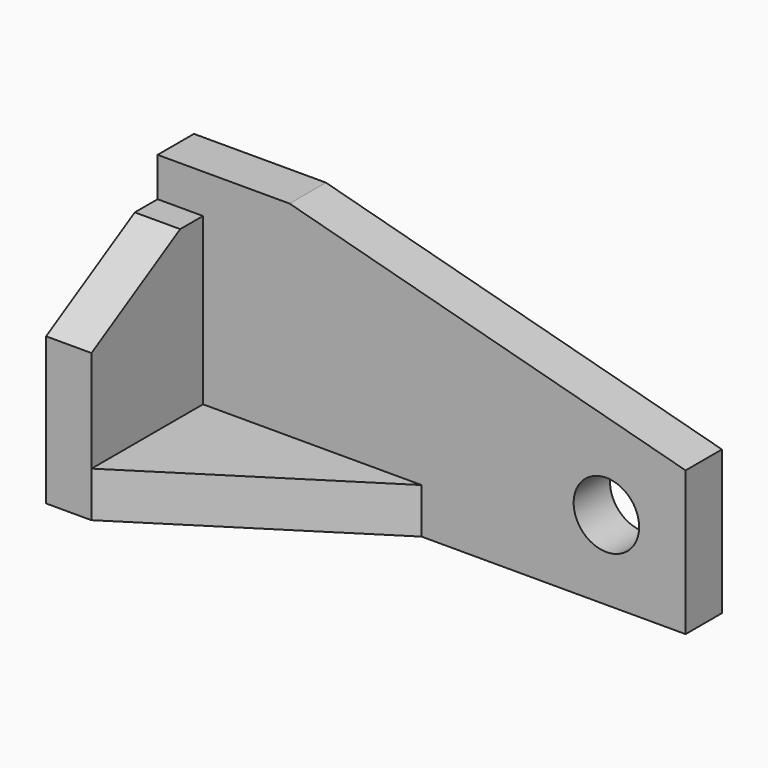
from build123d import *

# Parameters (mm, degrees)
F0_W     = 10.922
F0_H     = 28.702
F0_W_2   = 52.578
F0_H_2   = 10.922
F0_R     = 7.874
F1_DEPTH = 10.922
F2_DEPTH = 44.45
F3_SIZE2 = 52.628408
F3_SIZE  = 33.52799
F4_SIZE2 = 15.3979316793
F4_SIZE  = 26.67


# Not quite as in the source:
# - a fillet or chamfer is up to 0.001 mm smaller than in the source, because OpenCascade refuses the exact size


with BuildPart() as f1:
    # F0 (on Front) → F1 (new body)
    with BuildSketch(Plane.XZ):
        with Locations((-40.1902680954, 6.35)):
            Rectangle(F0_W, F0_H)
        with Locations((-8.4402680954, -24.638)):
            Rectangle(F0_W_2, F0_H_2)
        Polygon((-13.9012680954, 30.099), (-45.6512680954, 30.099), (-45.6512680954, 20.701), (-34.7292680954, 20.701), (-34.7292680954, -8.001), (-34.7292680954, -19.177), (17.8487319046, -19.177), (17.8487319046, -30.099), (81.3487319046, -30.099), (81.3487319046, 4.5768394209), align=None)
        with Locations((62.2987319046, -11.049)):
            Circle(F0_R, mode=Mode.SUBTRACT)
        Polygon((-34.7292680954, -8.001), (-45.6512680954, -8.001), (-45.6512680954, -30.099), (-34.7292680954, -30.099), (-34.7292680954, -19.177), align=None)
    extrude(amount=F1_DEPTH)

    # F0 (on Front) → F2 (join)
    with BuildSketch(Plane.XZ):
        with Locations((-40.1902680954, 6.35)):
            Rectangle(F0_W, F0_H)
        with Locations((-8.4402680954, -24.638)):
            Rectangle(F0_W_2, F0_H_2)
        Polygon((-34.7292680954, -8.001), (-45.6512680954, -8.001), (-45.6512680954, -30.099), (-34.7292680954, -30.099), (-34.7292680954, -19.177), align=None)
    extrude(amount=F2_DEPTH)

    # F3 (size 33.528 and 52.6284180296 in the source; OpenCascade refuses exactly that, so slightly less here)
    f3_edges = [f1.edges().sort_by_distance(p)[0] for p in [
        (17.848732, -44.45, -24.638),
    ]]
    f3_side = f1.faces().sort_by_distance((17.848732, -27.686, -24.638))[0]
    chamfer(f3_edges, length=F3_SIZE, length2=F3_SIZE2, reference=f3_side)

    # F4
    f4_edges = [f1.edges().sort_by_distance(p)[0] for p in [
        (-40.215472, -44.45, 20.701),
    ]]
    f4_side = f1.faces().sort_by_distance((-40.19028, -27.685963, 20.701))[0]
    chamfer(f4_edges, length=F4_SIZE, length2=F4_SIZE2, reference=f4_side)


solid = f1.part
